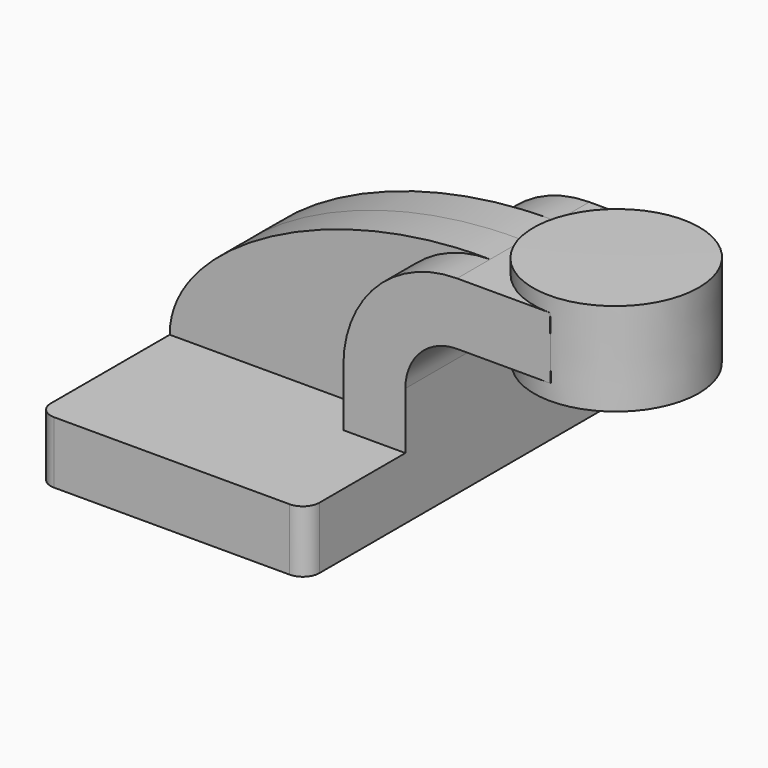
from build123d import *

# Parameters (mm, degrees)
F1_DEPTH = 63.5
F2_DEPTH = 25.4
F3_R     = 5.08
F4_DEPTH = 12.7


with BuildPart() as f1:
    # F0 (on Front) → F1 (new body, symmetric)
    with BuildSketch(Plane.XZ):
        Polygon((41.275, -9.525), (41.275, 9.525), (22.225, 9.525), (-41.275, 9.525), (-41.275, -9.525), align=None)
    extrude(amount=F1_DEPTH, both=True)

    # F0 (on Front) → F2 (join, symmetric)
    with BuildSketch(Plane.XZ):
        Polygon((60.325, 61.9252), (60.325, 42.8752), (85.8628631749, 42.8752), (85.752513782, 61.9252), align=None)
        with BuildLine():
            Line((22.225, 9.525), (41.275, 9.525))
            Line((41.275, 9.525), (41.275, 27.0002))
            ThreePointArc((41.275, 27.0002), (45.9246798487, 38.2255201513), (57.15, 42.8752))
            Line((57.15, 42.8752), (60.325, 42.8752))
            Line((60.325, 42.8752), (60.325, 61.9252))
            Line((60.325, 61.9252), (57.15, 61.9252))
            ThreePointArc((57.15, 61.9252), (32.4542956671, 51.6959043329), (22.225, 27.0002))
            Line((22.225, 27.0002), (22.225, 9.525))
        make_face()
    extrude(amount=F2_DEPTH, both=True)

    # F3
    f3_edges = [f1.edges().sort_by_distance(p)[0] for p in [
        (-41.275, -63.5, 0),
        (41.275, -63.5, 0),
        (41.275, 63.5, 0),
        (-41.275, 63.5, 0),
    ]]
    fillet(f3_edges, radius=F3_R)

    # F0 (on Front) → F4 (join, symmetric)
    with BuildSketch(Plane.XZ):
        Polygon((41.275, -9.525), (41.275, 9.525), (22.225, 9.525), (-41.275, 9.525), (-41.275, -9.525), align=None)
        with BuildLine():
            Line((-41.275, 9.525), (22.225, 9.525))
            Line((22.225, 9.525), (22.225, 27.0002))
            ThreePointArc((22.225, 27.0002), (32.4542956671, 51.6959043329), (57.15, 61.9252))
            add(Edge.make_bspline(
                [(-41.275, 9.525), (-41.4384305477, 35.2854393423), (6.2785348855, 62.6599118114), (57.15, 61.9252)],
                knots=[0, 0, 0, 0, 111.5045361635, 111.5045361635, 111.5045361635, 111.5045361635], degree=3))
        make_face()
        Polygon((85.8628631749, 42.8752), (60.325, 42.8752), (60.325, 38.1), (85.8905240893, 38.1), align=None)
        with BuildLine():
            Line((22.225, 9.525), (41.275, 9.525))
            Line((41.275, 9.525), (41.275, 27.0002))
            ThreePointArc((41.275, 27.0002), (45.9246798487, 38.2255201513), (57.15, 42.8752))
            Line((57.15, 42.8752), (60.325, 42.8752))
            Line((60.325, 42.8752), (60.325, 61.9252))
            Line((60.325, 61.9252), (57.15, 61.9252))
            ThreePointArc((57.15, 61.9252), (32.4542956671, 51.6959043329), (22.225, 27.0002))
            Line((22.225, 27.0002), (22.225, 9.525))
        make_face()
        Polygon((60.325, 61.9252), (60.325, 42.8752), (85.8628631749, 42.8752), (85.752513782, 61.9252), align=None)
    extrude(amount=F4_DEPTH, both=True)

    # F0 (on Front) → F5 (revolve)
    with BuildSketch(Plane.XZ):
        Polygon((85.752513782, 61.9252), (85.8628631749, 42.8752), (85.8905240893, 38.1), (111.125, 38.1), (111.125, 66.675), (85.725, 66.675), align=None)
    revolve(axis=Axis((85.8077620447, 0, 52.3875), (0.0057925219, 0, -0.9999832232)))


solid = f1.part
